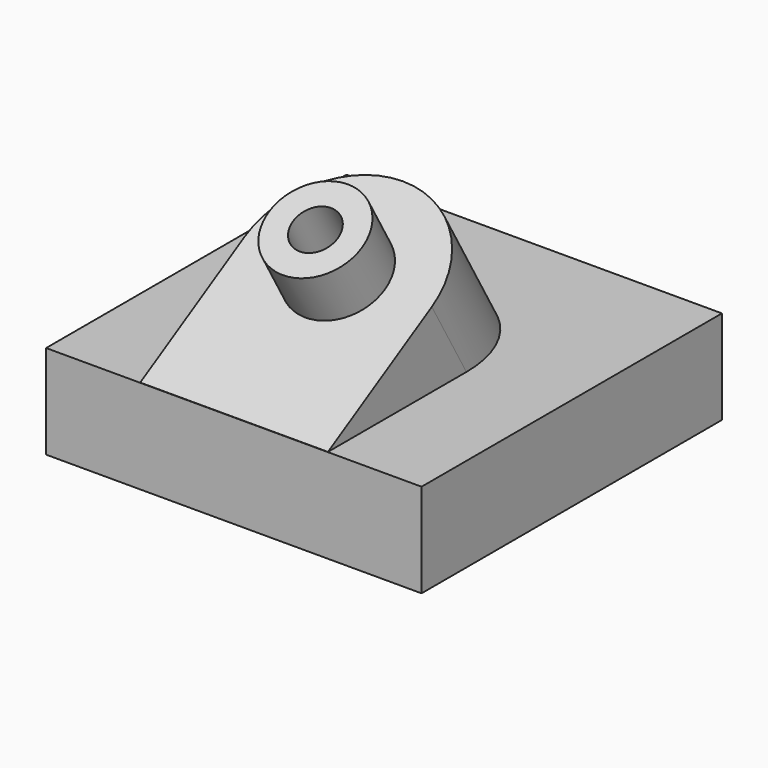
from build123d import *

# Parameters (mm, degrees)
F0_W      = 100
F0_H      = 25
F1_DEPTH  = 100
F7_W      = 50
F7_H      = 40
F8_R      = 25
F9_R      = 12.5
F12_DEPTH = 15
F13_R     = 6
F14_REACH = 55.0172779755


with BuildPart() as f1:
    # F0 (on Front) → F1 (new body)
    with BuildSketch(Plane.XZ):
        with Locations((50, -12.5)):
            Rectangle(F0_W, F0_H)
    extrude(amount=F1_DEPTH)

    # F7 (on line) + F8 (on line) → F11 (join, up to the next surface of F1)
    with BuildSketch(Plane(origin=(0, -24.9763522297, 43.2603110496), x_dir=(1, 0, 0), z_dir=(0, -0.5, 0.8660254038))):
        with Locations((50, -66.6025403784)):
            Rectangle(F7_W, F7_H)
    with BuildSketch(Plane(origin=(0, -24.9763522297, 43.2603110496), x_dir=(1, 0, 0), z_dir=(0, -0.5, 0.8660254038))):
        with Locations((50, -46.6025403784)):
            Circle(F8_R)
    extrude(until=Until.NEXT, dir=(0, 0.5, -0.8660254038))

    # F9 (on line) → F12 (join)
    with BuildSketch(Plane(origin=(0, -24.9763522297, 43.2603110496), x_dir=(1, 0, 0), z_dir=(0, -0.5, 0.8660254038))):
        with Locations((50, -46.6025403784)):
            Circle(F9_R)
    extrude(amount=F12_DEPTH)

    f14_end = Plane.XY
    # F13 (on face) → F14 (cut, up to a plane its end follows)
    with BuildSketch(Plane(origin=(0, -32.4763522297, 56.2506921064), x_dir=(1, 0, 0), z_dir=(0, -0.5, 0.8660254038))):
        with Locations((50, -46.6025403784)):
            Circle(F13_R)
    f14_long = extrude(amount=-F14_REACH, mode=Mode.PRIVATE)
    add(split(f14_long, bisect_by=f14_end, keep=Keep.TOP, mode=Mode.PRIVATE), mode=Mode.SUBTRACT)


solid = f1.part
